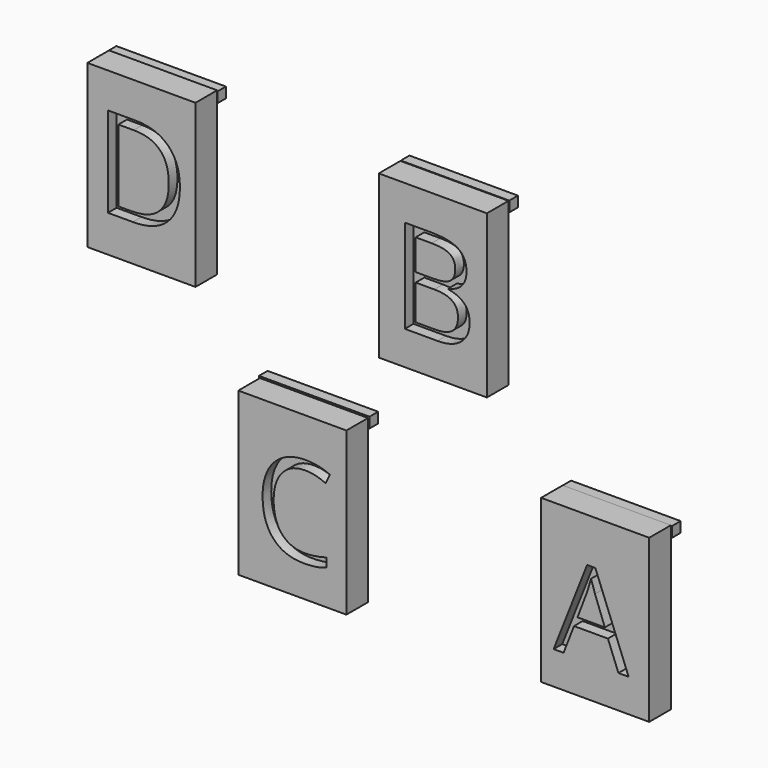
from build123d import *

# Parameters (mm, degrees)
F0_W           = 25.4
F0_H           = 38.1
F1_DEPTH       = 6.35
F2_R           = 3.81
F3_DEPTH       = 2.54
F5_TEXT_SIZE   = 27.849452777
F5_TEXT_SIZE_2 = 30.7809768452
F5_TEXT_SIZE_3 = 29.3152096371
F5_TEXT_SIZE_4 = 29.6816540261
F6_DEPTH       = 25.4
F7_W           = 25.730624795
F7_H           = 2.4505369365
F8_DEPTH       = 2.54
F7_W_2         = 25.4855751991
F7_W_3         = 25.7306285203
F7_W_4         = 25.9756827727
F7_H_2         = 2.4505350739


# Not quite as in the source:
# - Text() gives the source's letters only with a copy of the font that has no kerning and outlines rounded to 1/6400 em; it was checked with that copy


with BuildPart() as f1:
    # F0 (on Front) → F1 (new body)
    with BuildSketch(Plane.XZ):
        with Locations((-46.0602159804, 19.2970331914)):
            Rectangle(F0_W, F0_H)
    extrude(amount=F1_DEPTH)

    # F2 (on Front) → F3, piece 4 (join)
    with BuildSketch(Plane.XZ):
        with Locations((-40.9802159804, 28.1870331914)):
            Circle(F2_R)
        with Locations((-51.1402159804, 28.1870331914)):
            Circle(F2_R)
        with Locations((-51.1402159804, 18.0270331914)):
            Circle(F2_R)
    extrude(amount=-F3_DEPTH)


with BuildPart() as f1b:
    # F0 (on Front) → F1, piece 2 (new body)
    with BuildSketch(Plane.XZ):
        with Locations((-10.603061258, -36.9614025138)):
            Rectangle(F0_W, F0_H)
    extrude(amount=F1_DEPTH)

    # F2 (on Front) → F3, piece 2 (join)
    with BuildSketch(Plane.XZ):
        with Locations((-5.523061258, -28.0714025138)):
            Circle(F2_R)
        with Locations((-15.683061258, -28.0714025138)):
            Circle(F2_R)
    extrude(amount=-F3_DEPTH)


with BuildPart() as f1c:
    # F0 (on Front) → F1, piece 3 (new body)
    with BuildSketch(Plane.XZ):
        with Locations((60.5514380593, -36.0065931796)):
            Rectangle(F0_W, F0_H)
    extrude(amount=F1_DEPTH)

    # F2 (on Front) → F3 (join)
    with BuildSketch(Plane.XZ):
        with Locations((65.6314380593, -27.1165931796)):
            Circle(F2_R)
    extrude(amount=-F3_DEPTH)


with BuildPart() as f1d:
    # F0 (on Front) → F1, piece 4 (new body)
    with BuildSketch(Plane.XZ):
        with Locations((22.4085926682, 18.6961098781)):
            Rectangle(F0_W, F0_H)
    extrude(amount=F1_DEPTH)

    # F2 (on Front) → F3, piece 3 (join)
    with BuildSketch(Plane.XZ):
        with Locations((27.4885926682, 17.4261098781)):
            Circle(F2_R)
        with Locations((27.4885926682, 27.5861098781)):
            Circle(F2_R)
    extrude(amount=-F3_DEPTH)


with BuildPart() as f6_tool:
    # F5 (on offset) → F6 (new body)
    with BuildSketch(Plane.XZ.offset(3.81)):
        with Locations((50.7924966514, -47.2972951829)):
            Text('A', F5_TEXT_SIZE, font='Open Sans', text_align=(TextAlign.LEFT, TextAlign.BOTTOM))
        with Locations((12.8000043333, 7.5807813555)):
            Text('B', F5_TEXT_SIZE_2, font='Open Sans', text_align=(TextAlign.LEFT, TextAlign.BOTTOM))
        with Locations((-19.3881038576, -48.3526401222)):
            Text('C', F5_TEXT_SIZE_3, font='Open Sans', text_align=(TextAlign.LEFT, TextAlign.BOTTOM))
        with Locations((-56.8529367447, 8.8999718428)):
            Text('D', F5_TEXT_SIZE_4, font='Open Sans', text_align=(TextAlign.LEFT, TextAlign.BOTTOM))
    extrude(amount=F6_DEPTH)


with BuildPart() as f1_1:
    add(f1.part)

    # F6: cut by f6_tool
    add(f6_tool.part, mode=Mode.SUBTRACT)

    # F7 (on Front) → F8, piece 3 (join)
    with BuildSketch(Plane.XZ):
        with Locations((-46.1926031858, 36.8805658072)):
            Rectangle(F7_W_3, F7_H)
    extrude(amount=-F8_DEPTH)


with BuildPart() as f1b_1:
    add(f1b.part)

    # F6: cut by f6_tool
    add(f6_tool.part, mode=Mode.SUBTRACT)

    # F7 (on Front) → F8, piece 4 (join)
    with BuildSketch(Plane.XZ):
        with Locations((-10.5373053811, -18.7466004863)):
            Rectangle(F7_W_4, F7_H_2)
    extrude(amount=-F8_DEPTH)


with BuildPart() as f1c_1:
    add(f1c.part)

    # F6: cut by f6_tool
    add(f6_tool.part, mode=Mode.SUBTRACT)

    # F7 (on Front) → F8 (join)
    with BuildSketch(Plane.XZ):
        with Locations((60.6507658958, -18.2564929128)):
            Rectangle(F7_W, F7_H)
    extrude(amount=-F8_DEPTH)


with BuildPart() as f1d_1:
    add(f1d.part)

    # F6: cut by f6_tool
    add(f6_tool.part, mode=Mode.SUBTRACT)

    # F7 (on Front) → F8, piece 2 (join)
    with BuildSketch(Plane.XZ):
        with Locations((22.5449316204, 36.6355124861)):
            Rectangle(F7_W_2, F7_H)
    extrude(amount=-F8_DEPTH)


solid = Compound([f1_1.part, f1b_1.part, f1c_1.part, f1d_1.part])
